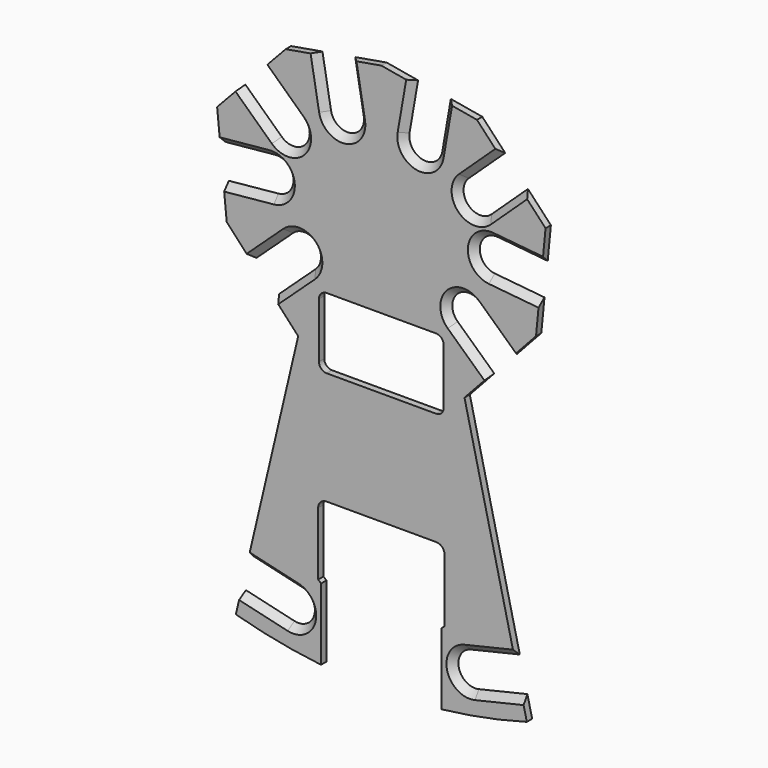
from build123d import *

# Parameters (mm, degrees)
F1_DEPTH = 8


# Not quite as in the source:
# - ends of sketch curves that miss each other by under 0.0002 mm in the source are joined


with BuildPart() as f1:
    # F0 (on Front) → F1 (new body)
    with BuildSketch(Plane.XZ):
        with BuildLine():
            Line((76, -164), (76, -239.943211))
            Line((76, -239.943211), (72.5, -242.910554))
            Line((72.5, -242.910554), (72.5, -329))
            ThreePointArc((72.5, -329), (124.1533829832, -321.067337789), (175.0000000351, -309.0000001251))
            Line((175.0000000351, -309.0000001251), (169.278269, -284.66357))
            Line((169.278269, -284.66357), (110.870838, -298.395725))
            ThreePointArc((110.870838, -298.395725), (86.8243094388, -283.5039655144), (101.716068848, -259.4574373536))
            Line((101.716068848, -259.4574373536), (160.123499, -245.725283))
            Line((160.123499, -245.725283), (100, 10))
            Line((100, 10), (129.421287, 41.816044))
            Line((129.421287, 41.816044), (85.369419, 82.552181))
            ThreePointArc((85.369419, 82.552181), (84.2641744646, 110.8148490327), (112.5268427835, 111.9200937658))
            Line((112.5268427835, 111.9200937658), (156.578712, 71.183957))
            Line((156.578712, 71.183957), (186, 103))
            Line((186, 103), (189.810038, 142.094309))
            Line((189.810038, 142.094309), (130.092964, 147.914193))
            ThreePointArc((130.092964, 147.914193), (112.1272346173, 169.7598464886), (133.9728870415, 187.7255764263))
            Line((133.9728870415, 187.7255764263), (193.689961, 181.905692))
            Line((193.689961, 181.905692), (197.5, 221))
            Line((197.5, 221), (169.928822, 250.409256))
            Line((169.928822, 250.409256), (126.15659, 209.372789))
            ThreePointArc((126.15659, 209.372789), (97.8870239172, 210.2847104224), (98.7989451563, 238.5542768333))
            Line((98.7989451563, 238.5542768333), (142.571177, 279.590745))
            Line((142.571177, 279.590745), (115, 309))
            Line((115, 309), (77.204235, 315.573177))
            Line((77.204235, 315.573177), (66.923764, 256.460472))
            ThreePointArc((66.923764, 256.460472), (43.7927054839, 240.1830599073), (27.5152939917, 263.3141190014))
            Line((27.5152939917, 263.3141190014), (37.795765, 322.426824))
            Line((37.795765, 322.426824), (0, 329))
            Line((0, 329), (-37.795765, 322.426824))
            Line((-37.795765, 322.426824), (-27.515295, 263.314119))
            ThreePointArc((-27.515295, 263.314119), (-43.7927064839, 240.1830599073), (-66.9237651771, 256.4604719692))
            Line((-66.9237651771, 256.4604719692), (-77.204235, 315.573177))
            Line((-77.204235, 315.573177), (-115, 309))
            Line((-115, 309), (-142.571178, 279.590745))
            Line((-142.571178, 279.590745), (-98.798945, 238.554277))
            ThreePointArc((-98.798945, 238.554277), (-97.8870241667, 210.2847101563), (-126.1565908437, 209.3727891667))
            Line((-126.1565908437, 209.3727891667), (-169.928823, 250.409256))
            Line((-169.928823, 250.409256), (-197.5, 221))
            Line((-197.5, 221), (-193.689962, 181.905692))
            Line((-193.689962, 181.905692), (-133.972888, 187.725576))
            ThreePointArc((-133.972888, 187.725576), (-112.1272346173, 169.7598464886), (-130.092965055, 147.9141935643))
            Line((-130.092965055, 147.9141935643), (-189.810039, 142.094309))
            Line((-189.810039, 142.094309), (-186, 103))
            Line((-186, 103), (-156.578713, 71.183957))
            Line((-156.578713, 71.183957), (-112.526844, 111.920094))
            ThreePointArc((-112.526844, 111.920094), (-84.2641747139, 110.8148493022), (-85.3694187181, 82.5521806951))
            Line((-85.3694187181, 82.5521806951), (-129.421288, 41.816044))
            Line((-129.421288, 41.816044), (-100, 10))
            Line((-100, 10), (-160.1235, -245.725283))
            Line((-160.1235, -245.725283), (-101.716069, -259.457438))
            ThreePointArc((-101.716069, -259.457438), (-86.8243105502, -283.5039659882), (-110.8708388768, -298.395724476))
            Line((-110.8708388768, -298.395724476), (-169.278269, -284.66357))
            Line((-169.278269, -284.66357), (-175, -309))
            ThreePointArc((-175, -309), (-124.1533829832, -321.067337789), (-72.5000000145, -329.0000001291))
            Line((-72.5000000145, -329.0000001291), (-72.5, -242.910554))
            Line((-72.5, -242.910554), (-76, -239.943211))
            Line((-76, -239.943211), (-76, -164))
            ThreePointArc((-76, -164), (-73.0710678119, -156.9289321881), (-66, -154))
            Line((-66, -154), (0, -154))
            Line((0, -154), (66, -154))
            ThreePointArc((66, -154), (73.0710678119, -156.9289321881), (76, -164))
        make_face()
        with BuildLine():
            Line((65.800007, -18.166468), (0, -18.166468))
            Line((0, -18.166468), (-65.800008, -18.166468))
            ThreePointArc((-65.800008, -18.166468), (-72.3053903869, -15.4718503869), (-75.000008, -8.966468))
            Line((-75.000008, -8.966468), (-75.000008, 57.633575))
            ThreePointArc((-75.000008, 57.633575), (-72.3053903869, 64.1389573869), (-65.800008, 66.833575))
            Line((-65.800008, 66.833575), (0, 66.833575))
            Line((0, 66.833575), (65.800007, 66.833575))
            ThreePointArc((65.800007, 66.833575), (72.3053893869, 64.1389573869), (75.000007, 57.633575))
            Line((75.000007, 57.633575), (75.000007, -8.966468))
            ThreePointArc((75.000007, -8.966468), (72.3053893869, -15.4718503869), (65.800007, -18.166468))
        make_face(mode=Mode.SUBTRACT)
    extrude(amount=F1_DEPTH)

    # F3: sweep along a path in F3_path
    with BuildLine(Plane(origin=(110.870838, -8, -298.395725), x_dir=(0, 0, 1), z_dir=(0, -1, 0))) as f3_path:
        Line((13.732155, -58.407431), (0, 0))
        ThreePointArc((0, 0), (14.8917592236, 24.0465284996), (38.9382876464, 9.154769152))
        Line((38.9382876464, 9.154769152), (52.670442, -49.252661))
    # F2 (on face) → F3 (sweep, cut)
    with BuildSketch(Plane(origin=(96.989833717, 0, 22.8032516792), x_dir=(0, 1, 0), z_dir=(0.973457176, 0, 0.2288692344))):
        Polygon((0, -315.8503827909), (-8, -315.8503827909), (-8, -323.8503827909), align=None)
    sweep(path=f3_path.line, mode=Mode.SUBTRACT)

    # F5: sweep along a path in F5_path
    with BuildLine(Plane(origin=(85.369419, -8, 82.552181), x_dir=(0, 0, 1), z_dir=(0, -1, 0))) as f5_path:
        Line((-40.736137, -44.051868), (0, 0))
        ThreePointArc((0, 0), (28.2626681852, 1.1052443944), (29.3679127658, -27.1574237835))
        Line((29.3679127658, -27.1574237835), (-11.368224, -71.209293))
    # F4 (on face) → F5 (sweep, cut)
    with BuildSketch(Plane(origin=(48.9199144477, 0, -45.2377688119), x_dir=(0, 1, 0), z_dir=(0.7341978267, 0, -0.6789356017))):
        Polygon((0, 118.5699679847), (-8, 118.5699679847), (-8, 110.5699679847), align=None)
    sweep(path=f5_path.line, mode=Mode.SUBTRACT)

    # F7: sweep along a path in F7_path
    with BuildLine(Plane(origin=(130.092964, -8, 147.914193), x_dir=(0, 0, 1), z_dir=(0, -1, 0))) as f7_path:
        Line((-5.819884, -59.717074), (0, 0))
        ThreePointArc((0, 0), (21.8456531581, 17.9657294149), (39.8113834263, -3.8799230415))
        Line((39.8113834263, -3.8799230415), (33.991499, -63.596997))
    # F6 (on face) → F7 (sweep, cut)
    with BuildSketch(Plane(origin=(174.3063070687, 0, -16.9874764527), x_dir=(0, 1, 0), z_dir=(0.9952845708, 0, -0.0969980576))):
        Polygon((0, 159.8354783382), (-8, 159.8354783382), (-8, 151.8354783382), align=None)
    sweep(path=f7_path.line, mode=Mode.SUBTRACT)

    # F9: sweep along a path in F9_path
    with BuildLine(Plane(origin=(126.15659, -8, 209.372789), x_dir=(0, 0, 1), z_dir=(0, -1, 0))) as f9_path:
        Line((41.036467, -43.772232), (0, 0))
        ThreePointArc((0, 0), (0.9119215885, 28.2695662386), (29.1814878333, 27.3576448437))
        Line((29.1814878333, 27.3576448437), (70.217956, -16.414587))
    # F8 (on face) → F9 (sweep, cut)
    with BuildSketch(Plane(origin=(215.3846137301, 0, 201.9230790338), x_dir=(0, 1, 0), z_dir=(0.729537198, 0, 0.6839411355))):
        Polygon((0, 66.4615554934), (-8, 66.4615554934), (-8, 58.4615554934), align=None)
    sweep(path=f9_path.line, mode=Mode.SUBTRACT)

    # F11: sweep along a path in F11_path
    with BuildLine(Plane(origin=(66.923764, -8, 256.460472), x_dir=(0, 0, 1), z_dir=(0, -1, 0))) as f11_path:
        Line((59.112705, -10.280471), (0, 0))
        ThreePointArc((0, 0), (-16.2774120773, 23.1310586047), (6.8536470014, 39.4084700083))
        Line((6.8536470014, 39.4084700083), (65.966352, 29.127999))
    # F10 (on face) → F11 (sweep, cut)
    with BuildSketch(Plane(origin=(55.5376187282, 0, 319.3412844519), x_dir=(0.9852117527, 0, -0.1713411869), z_dir=(0.1713411869, 0, 0.9852117527))):
        Polygon((21.9918369956, 0), (21.9918369956, -8), (29.9918369956, -8), align=None)
    sweep(path=f11_path.line, mode=Mode.SUBTRACT)

    # F13: sweep along a path in F13_path
    with BuildLine(Plane(origin=(-27.515295, -8, 263.314119), x_dir=(0, 0, 1), z_dir=(0, -1, 0))) as f13_path:
        Line((59.112705, 10.28047), (0, 0))
        ThreePointArc((0, 0), (-23.1310590934, 16.277411488), (-6.8536470308, 39.4084701771))
        Line((-6.8536470308, 39.4084701771), (52.259058, 49.68894))
    # F12 (on face) → F13 (sweep, cut)
    with BuildSketch(Plane(origin=(-55.5376105295, 0, 319.341285892), x_dir=(0.9852117571, 0, 0.1713411616), z_dir=(-0.1713411616, 0, 0.9852117571))):
        Polygon((18.008154492, 0), (18.008154492, -8), (26.008154492, -8), align=None)
    sweep(path=f13_path.line, mode=Mode.SUBTRACT)

    # F15: sweep along a path in F15_path
    with BuildLine(Plane(origin=(-126.1565908437, -8, 209.3727891667), x_dir=(0, 0, -1), z_dir=(0, 1, 0))) as f15_path:
        Line((-41.0364668333, 43.7722321563), (0, 0))
        ThreePointArc((0, 0), (-0.9119210729, -28.2695667552), (-29.1814878333, -27.3576458437))
        Line((-29.1814878333, -27.3576458437), (-70.2179558333, 16.4145871563))
    # F14 (on face) → F15 (sweep, cut)
    with BuildSketch(Plane(origin=(-215.3846129172, 0, 201.9230851377), x_dir=(0, -1, 0), z_dir=(-0.7295371863, 0, 0.6839411479))):
        Polygon((0, 106.461550303), (8, 106.461550303), (8, 114.461550303), align=None)
    sweep(path=f15_path.line, mode=Mode.SUBTRACT)

    # F17: sweep along a path in F17_path
    with BuildLine(Plane(origin=(-133.972888, -8, 187.725576), x_dir=(0, 0, 1), z_dir=(0, -1, 0))) as f17_path:
        Line((-5.819884, 59.717074), (0, 0))
        ThreePointArc((0, 0), (-17.9657296763, -21.8456533988), (-39.8113824357, -3.879922945))
        Line((-39.8113824357, -3.879922945), (-45.631267, 55.837151))
    # F16 (on face) → F17 (sweep, cut)
    with BuildSketch(Plane(origin=(-174.3063082, 0, -16.9874769975), x_dir=(0, -1, 0), z_dir=(-0.9952845705, 0, -0.09699806))):
        Polygon((0, 199.8354791034), (8, 199.8354791034), (8, 207.8354791034), align=None)
    sweep(path=f17_path.line, mode=Mode.SUBTRACT)

    # F19: sweep along a path in F19_path
    with BuildLine(Plane(origin=(-112.526844, -8, 111.920094), x_dir=(0, 0, 1), z_dir=(0, -1, 0))) as f19_path:
        Line((-40.736137, 44.051869), (0, 0))
        ThreePointArc((0, 0), (-1.1052443315, -28.2626689474), (-29.3679133049, -27.1574252819))
        Line((-29.3679133049, -27.1574252819), (-70.10405, 16.894444))
    # F18 (on face) → F19 (sweep, cut)
    with BuildSketch(Plane(origin=(-48.9199129921, 0, -45.2377688877), x_dir=(0, -1, 0), z_dir=(-0.7341978161, 0, -0.6789356132))):
        Polygon((0, 158.5699702901), (8, 158.5699702901), (8, 166.5699702901), align=None)
    sweep(path=f19_path.line, mode=Mode.SUBTRACT)

    # F21: sweep along a path in F21_path
    with BuildLine(Plane(origin=(-101.716069, -8, -259.457438), x_dir=(0, 0, 1), z_dir=(0, -1, 0))) as f21_path:
        Line((13.732155, 58.407431), (0, 0))
        ThreePointArc((0, 0), (-24.0465282, -14.8917584), (-38.938286476, 9.1547698768))
        Line((-38.938286476, 9.1547698768), (-25.206132, 67.5622))
    # F20 (on face) → F21 (sweep, cut)
    with BuildSketch(Plane(origin=(-96.9898309629, 0, 22.8032521208), x_dir=(0, -1, 0), z_dir=(-0.9734571736, 0, 0.2288692447))):
        Polygon((0, -275.8503839769), (8, -275.8503839769), (8, -267.8503839769), align=None)
    sweep(path=f21_path.line, mode=Mode.SUBTRACT)


solid = f1.part
